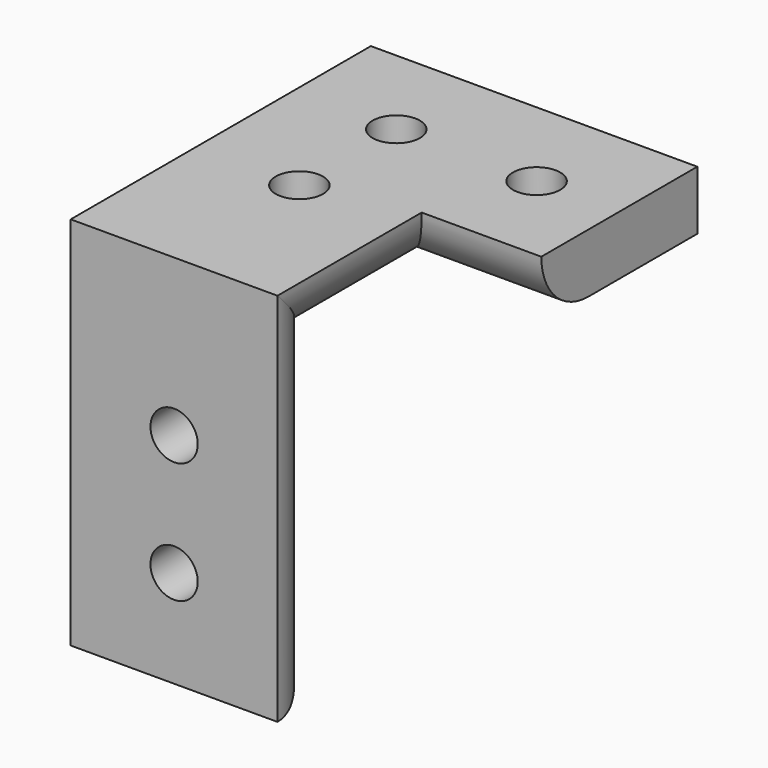
from build123d import *

# Parameters (mm, degrees)
F0_R     = 1.6
F1_DEPTH = 4
F0_W     = 14
F0_H     = 4
F2_DEPTH = 25.4
F3_R     = 1.6
F4_DEPTH = 4
F5_R     = 3.99999


# Not quite as in the source:
# - a fillet or chamfer is up to 0.001 mm smaller than in the source, because OpenCascade refuses the exact size


with BuildPart() as f1:
    # F0 (on Top) → F1 (new body)
    with BuildSketch(Plane.XY):
        Polygon((7, 12.7), (-7, 12.7), (-7, -8.7), (7, -8.7), (7, -0.5), (15.1, -0.5), (15.1, 12.7), align=None)
        with Locations((0, -2.1)):
            Circle(F0_R, mode=Mode.SUBTRACT)
        with Locations((0, 6.1)):
            Circle(F0_R, mode=Mode.SUBTRACT)
        with Locations((9.5, 6.1)):
            Circle(F0_R, mode=Mode.SUBTRACT)
    extrude(amount=-F1_DEPTH)

    # F0 (on Top) → F2 (join)
    with BuildSketch(Plane.XY):
        with Locations((0, -10.7)):
            Rectangle(F0_W, F0_H)
    extrude(amount=-F2_DEPTH)

    # F3 (on face) → F4 (cut, through all)
    with BuildSketch(Plane(origin=(0, -8.7, 0), x_dir=(-1, 0, 0), z_dir=(0, 1, 0))):
        with Locations((0, -10.6)):
            Circle(F3_R)
        with Locations((0, -18.8)):
            Circle(F3_R)
    extrude(amount=-F4_DEPTH, mode=Mode.SUBTRACT)

    # F5 (radius 4 in the source; OpenCascade refuses exactly that, so slightly less here)
    f5_edges = [f1.edges().sort_by_distance(p)[0] for p in [
        (-7, -8.7, -14.7),
        (0, -8.7, -25.4),
        (7, -8.7, -14.7),
        (-7, 2, -4),
        (7, -4.6, -4),
        (11.05, -0.5, -4),
    ]]
    fillet(f5_edges, radius=F5_R)


solid = f1.part
